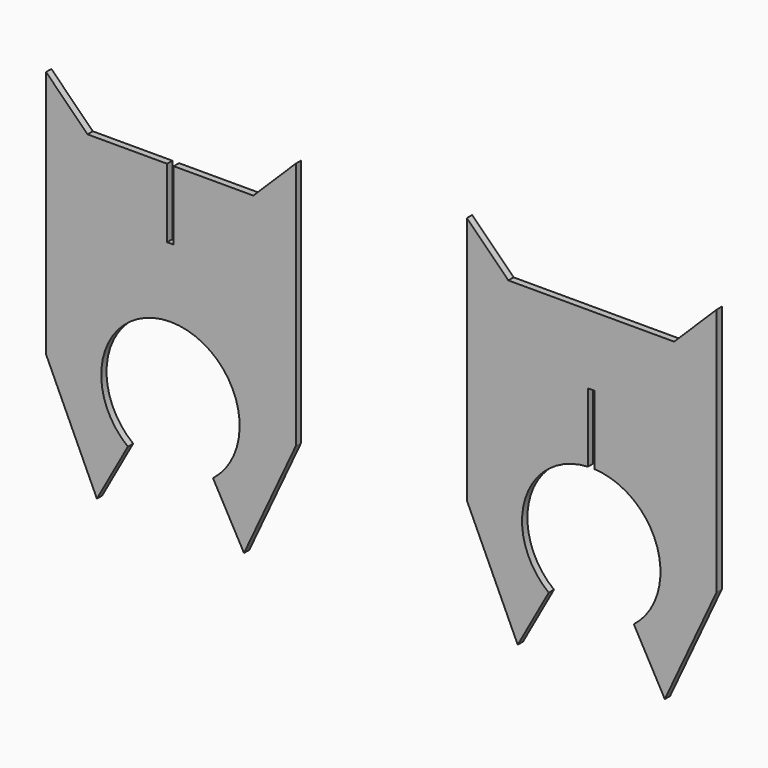
from build123d import *

# Parameters (mm, degrees)
F1_DEPTH = 1.524


# Not quite as in the source:
# - a feature names something its author has since deleted; it is built from what else it names


with BuildPart() as f1:
    # F0 (on Front) → F1 (new body)
    with BuildSketch(Plane.XZ):
        with BuildLine():
            ThreePointArc((-399.8226737201, -0.736120695), (-390.0420399189, 27.705359182), (-380.2614061177, -0.736120695))
            Line((-380.2614061177, -0.736120695), (-373.1401919201, -13.583131183))
            Line((-373.1401919201, -13.583131183), (-361.2339419201, 11.9302616742))
            Line((-361.2339419201, 11.9302616742), (-361.2339419201, 59.5552616742))
            Line((-361.2339419201, 59.5552616742), (-361.2339419201, 69.0802616742))
            Line((-361.2339419201, 69.0802616742), (-370.9920399189, 59.4279065132))
            Line((-370.9920399189, 59.4279065132), (-389.2800399189, 59.4279065132))
            Line((-389.2800399189, 59.4279065132), (-389.2800399189, 43.5529065132))
            Line((-389.2800399189, 43.5529065132), (-390.0420399189, 43.5529065132))
            Line((-390.0420399189, 43.5529065132), (-390.8040399189, 43.5529065132))
            Line((-390.8040399189, 43.5529065132), (-390.8040399189, 59.4279065132))
            Line((-390.8040399189, 59.4279065132), (-409.0920399189, 59.4279065132))
            Line((-409.0920399189, 59.4279065132), (-418.6170399189, 68.9529065132))
            Line((-418.6170399189, 68.9529065132), (-418.6170399189, 59.4279065132))
            Line((-418.6170399189, 59.4279065132), (-418.6170399189, 11.8029065132))
            Line((-418.6170399189, 11.8029065132), (-406.9438879177, -13.583131183))
            Line((-406.9438879177, -13.583131183), (-399.8226737201, -0.736120695))
        make_face()
    extrude(amount=F1_DEPTH)


with BuildPart() as f1b:
    # F0 (on Front) → F1, piece 2 (new body)
    with BuildSketch(Plane.XZ):
        with BuildLine():
            ThreePointArc((-292.5745729645, 29.5862229522), (-278.1788508217, 18.5115548851), (-283.5559391633, 1.1630099959))
            Line((-283.5559391633, 1.1630099959), (-276.4347249657, -11.6840004921))
            Line((-276.4347249657, -11.6840004921), (-264.5284749657, 13.8293923651))
            Line((-264.5284749657, 13.8293923651), (-264.5284749657, 61.4543923651))
            Line((-264.5284749657, 61.4543923651), (-264.5284749657, 70.9793923651))
            Line((-264.5284749657, 70.9793923651), (-274.2865729645, 61.3270372041))
            Line((-274.2865729645, 61.3270372041), (-312.3865729645, 61.3270372041))
            Line((-312.3865729645, 61.3270372041), (-321.9115729645, 70.8520372041))
            Line((-321.9115729645, 70.8520372041), (-321.9115729645, 61.3270372041))
            Line((-321.9115729645, 61.3270372041), (-321.9115729645, 13.7020372041))
            Line((-321.9115729645, 13.7020372041), (-310.2384209633, -11.6840004921))
            Line((-310.2384209633, -11.6840004921), (-303.1172067657, 1.1630099959))
            ThreePointArc((-303.1172067657, 1.1630099959), (-308.4942951073, 18.5115548851), (-294.0985729645, 29.5862229522))
            Line((-294.0985729645, 29.5862229522), (-294.0985729645, 45.4520372041))
            Line((-294.0985729645, 45.4520372041), (-293.3365729645, 45.4520372041))
            Line((-293.3365729645, 45.4520372041), (-292.5745729645, 45.4520372041))
            Line((-292.5745729645, 45.4520372041), (-292.5745729645, 29.5862229522))
        make_face()
    extrude(amount=F1_DEPTH)


solid = Compound([f1.part, f1b.part])
